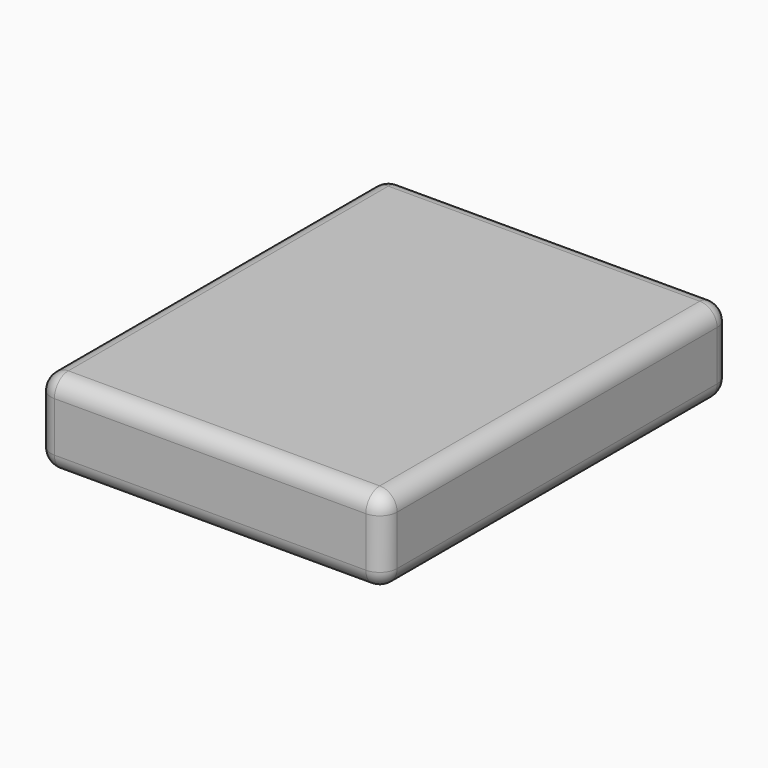
from build123d import *

# Parameters (mm, degrees)
F0_W     = 101.1528596282
F0_H     = 24.6861185879
F1_DEPTH = 63.5
F2_R     = 5.08


# Not quite as in the source:
# - a feature names something its author has since deleted; it is built from what else it names


with BuildPart() as f1:
    # F0 (on Front) → F1 (new body, symmetric)
    with BuildSketch(Plane.XZ):
        Rectangle(F0_W, F0_H)
    extrude(amount=F1_DEPTH, both=True)

    # F2
    f2_edges = [f1.edges().sort_by_distance(p)[0] for p in [
        (0, -63.5, 12.343059),
        (-50.57643, -63.5, 0),
        (0, -63.5, -12.343059),
        (50.57643, -63.5, 0),
        (50.57643, 63.5, 0),
        (50.57643, 0, 12.343059),
        (50.57643, 0, -12.343059),
        (-50.57643, 0, 12.343059),
        (-50.57643, 63.5, 0),
        (-50.57643, 0, -12.343059),
        (0, 63.5, 12.343059),
        (0, 63.5, -12.343059),
    ]]
    fillet(f2_edges, radius=F2_R)


solid = f1.part
